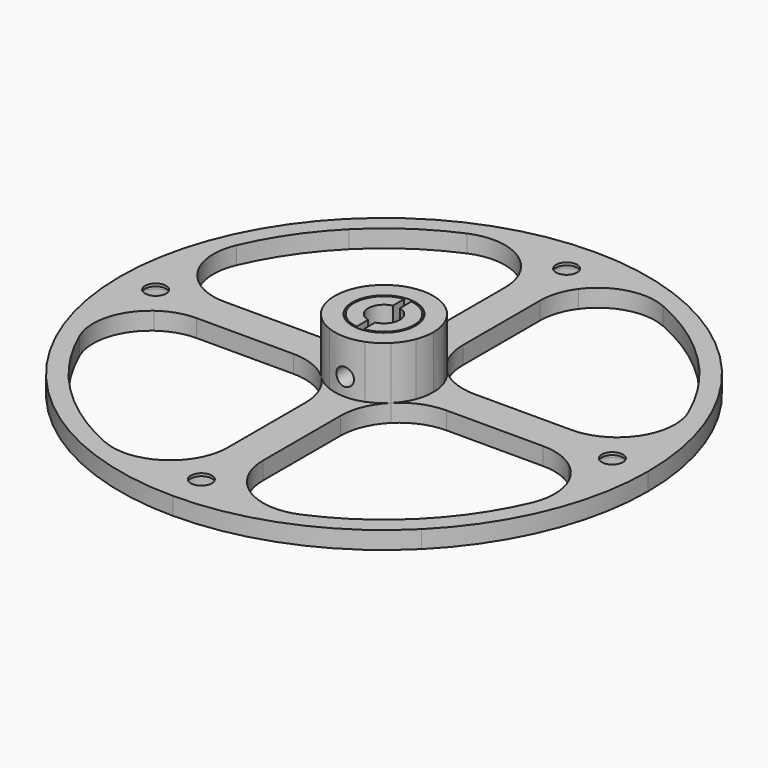
from build123d import *

# Parameters (mm, degrees)
F3_R          = 1.2
F3_R_2        = 2.05
F4_DEPTH      = 1
F4_DEPTH_BACK = 1
F5_DEPTH      = 1
F5_DEPTH_BACK = 1
F6_DEPTH      = 7
F7_DEPTH      = 0.7
F7_DEPTH_BACK = 0.7
F8_R          = 1
F9_DEPTH      = 30
F9_DEPTH_BACK = 30
F11_DEPTH     = 8


with BuildPart() as f4:
    # F3 (on Top) → F4 (new body, two sides)
    with BuildSketch(Plane.XY) as f4_sk:
        with BuildLine():
            Line((-19.79899, 19.79899), (-21.213203, 21.213203))
            ThreePointArc((-21.213203, 21.213203), (-27.716386, 11.480503), (-30, 0))
            ThreePointArc((-30, 0), (-29.396228, 2.127442), (-27.764933, 3.620569))
            ThreePointArc((-27.764933, 3.620569), (-26.989532, 7.454205), (-25.687491, 11.142389))
            ThreePointArc((-25.687491, 11.142389), (-23.15144, 15.74836), (-19.79899, 19.79899))
        make_face()
        with BuildLine():
            ThreePointArc((-30, 0), (-27.716386, -11.480503), (-21.213203, -21.213203))
            Line((-21.213203, -21.213203), (-19.79899, -19.79899))
            ThreePointArc((-19.79899, -19.79899), (-23.15144, -15.74836), (-25.687491, -11.142389))
            ThreePointArc((-25.687491, -11.142389), (-26.989532, -7.454205), (-27.764933, -3.620569))
            ThreePointArc((-27.764933, -3.620569), (-29.396228, -2.127443), (-30, 0))
        make_face()
        with BuildLine():
            ThreePointArc((-23.555055, -3.265997), (-25.610097, -4.035711), (-27.764933, -3.620569))
            ThreePointArc((-27.764933, -3.620569), (-26.989532, -7.454205), (-25.687491, -11.142389))
            ThreePointArc((-25.687491, -11.142389), (-26.000354, -6.830824), (-23.555055, -3.265997))
        make_face()
        with BuildLine():
            Line((-19.687728, 2), (-22.428282, 2))
            ThreePointArc((-22.428282, 2), (-22.034297, 1.034297), (-21.9, 0))
            ThreePointArc((-21.9, 0), (-22.034297, -1.034297), (-22.428282, -2))
            Line((-22.428282, -2), (-19.687728, -2))
            Line((-19.687728, -2), (-8.691169, -2))
            Line((-8.691169, -2), (-5.230679, -2))
            ThreePointArc((-5.230679, -2), (-5.6, 0), (-5.230679, 2))
            Line((-5.230679, 2), (-8.691169, 2))
            Line((-8.691169, 2), (-19.687728, 2))
        make_face()
        with BuildLine():
            ThreePointArc((22.428282, -2), (21.9, 0), (22.428282, 2))
            Line((22.428282, 2), (19.687728, 2))
            Line((19.687728, 2), (8.691169, 2))
            Line((8.691169, 2), (5.230679, 2))
            ThreePointArc((5.230679, 2), (5.506896, 1.016907), (5.6, 0))
            ThreePointArc((5.6, 0), (5.506896, -1.016907), (5.230679, -2))
            Line((5.230679, -2), (8.691169, -2))
            Line((8.691169, -2), (19.687728, -2))
            Line((19.687728, -2), (22.428282, -2))
        make_face()
        with BuildLine():
            Line((-2, -8.691169), (-2, -19.687728))
            Line((-2, -19.687728), (-2, -22.428282))
            ThreePointArc((-2, -22.428282), (0, -21.9), (2, -22.428282))
            Line((2, -22.428282), (2, -19.687728))
            Line((2, -19.687728), (2, -8.691169))
            Line((2, -8.691169), (2, -5.230679))
            ThreePointArc((2, -5.230679), (0, -5.6), (-2, -5.230679))
            Line((-2, -5.230679), (-2, -8.691169))
        make_face()
        with BuildLine():
            ThreePointArc((2, 22.428282), (0, 21.9), (-2, 22.428282))
            Line((-2, 22.428282), (-2, 19.687728))
            Line((-2, 19.687728), (-2, 8.691169))
            Line((-2, 8.691169), (-2, 5.230679))
            ThreePointArc((-2, 5.230679), (0, 5.6), (2, 5.230679))
            Line((2, 5.230679), (2, 8.691169))
            Line((2, 8.691169), (2, 19.687728))
            Line((2, 19.687728), (2, 22.428282))
        make_face()
        with BuildLine():
            ThreePointArc((-3.620569, 27.764933), (-2.127442, 29.396228), (0, 30))
            ThreePointArc((0, 30), (-11.480503, 27.716386), (-21.213203, 21.213203))
            Line((-21.213203, 21.213203), (-19.79899, 19.79899))
            ThreePointArc((-19.79899, 19.79899), (-15.74836, 23.15144), (-11.142389, 25.687491))
            ThreePointArc((-11.142389, 25.687491), (-7.454205, 26.989532), (-3.620569, 27.764933))
        make_face()
        with BuildLine():
            Line((19.79899, 19.79899), (21.213203, 21.213203))
            ThreePointArc((21.213203, 21.213203), (11.480503, 27.716386), (0, 30))
            ThreePointArc((0, 30), (2.127442, 29.396228), (3.620569, 27.764933))
            ThreePointArc((3.620569, 27.764933), (7.454205, 26.989532), (11.142389, 25.687491))
            ThreePointArc((11.142389, 25.687491), (15.74836, 23.15144), (19.79899, 19.79899))
        make_face()
        with BuildLine():
            ThreePointArc((3.620569, 27.764933), (2.127442, 29.396228), (0, 30))
            ThreePointArc((0, 30), (-2.127442, 29.396228), (-3.620569, 27.764933))
            ThreePointArc((-3.620569, 27.764933), (-1.814096, 27.941171), (0, 28))
            ThreePointArc((0, 28), (1.814096, 27.941171), (3.620569, 27.764933))
        make_face()
        with BuildLine():
            ThreePointArc((4.05, 25.95), (3.94118, 26.882522), (3.620569, 27.764933))
            ThreePointArc((3.620569, 27.764933), (1.814096, 27.941171), (0, 28))
            ThreePointArc((0, 28), (-1.814096, 27.941171), (-3.620569, 27.764933))
            ThreePointArc((-3.620569, 27.764933), (-4.035711, 25.610097), (-3.265997, 23.555055))
            ThreePointArc((-3.265997, 23.555055), (-2.692599, 22.924704), (-2, 22.428282))
            ThreePointArc((-2, 22.428282), (0, 21.9), (2, 22.428282))
            ThreePointArc((2, 22.428282), (2.692599, 22.924704), (3.265997, 23.555055))
            ThreePointArc((3.265997, 23.555055), (3.849012, 24.689998), (4.05, 25.95))
        make_face()
        with BuildLine():
            ThreePointArc((2.05, 25.95), (-1.449569, 24.500431), (0, 28))
            ThreePointArc((0, 28), (1.449569, 27.399569), (2.05, 25.95))
        make_face(mode=Mode.SUBTRACT)
        with BuildLine():
            ThreePointArc((-23.555055, 3.265998), (-25.610097, 4.035711), (-27.764933, 3.620569))
            ThreePointArc((-27.764933, 3.620569), (-27.941171, 1.814096), (-28, 0))
            ThreePointArc((-28, 0), (-27.941171, -1.814096), (-27.764933, -3.620569))
            ThreePointArc((-27.764933, -3.620569), (-25.610097, -4.035711), (-23.555055, -3.265997))
            ThreePointArc((-23.555055, -3.265997), (-22.924704, -2.692599), (-22.428282, -2))
            ThreePointArc((-22.428282, -2), (-22.034297, -1.034297), (-21.9, 0))
            ThreePointArc((-21.9, 0), (-22.034297, 1.034297), (-22.428282, 2))
            ThreePointArc((-22.428282, 2), (-22.924705, 2.692599), (-23.555055, 3.265998))
        make_face()
        with BuildLine():
            ThreePointArc((-23.9, 0), (-25.95, -2.05), (-28, 0))
            ThreePointArc((-28, 0), (-25.95, 2.05), (-23.9, 0))
        make_face(mode=Mode.SUBTRACT)
        with BuildLine():
            ThreePointArc((-27.764933, 3.620569), (-29.396228, 2.127442), (-30, 0))
            ThreePointArc((-30, 0), (-29.396228, -2.127443), (-27.764933, -3.620569))
            ThreePointArc((-27.764933, -3.620569), (-27.941171, -1.814096), (-28, 0))
            ThreePointArc((-28, 0), (-27.941171, 1.814096), (-27.764933, 3.620569))
        make_face()
        with BuildLine():
            ThreePointArc((-23.9, 0), (-25.95, 2.05), (-28, 0))
            ThreePointArc((-28, 0), (-25.95, -2.05), (-23.9, 0))
        make_face()
        with Locations((-25.95, 0)):
            Circle(F3_R, mode=Mode.SUBTRACT)
        with BuildLine():
            ThreePointArc((0, -30), (11.480503, -27.716386), (21.213203, -21.213203))
            Line((21.213203, -21.213203), (19.79899, -19.79899))
            ThreePointArc((19.79899, -19.79899), (15.74836, -23.15144), (11.142389, -25.687491))
            ThreePointArc((11.142389, -25.687491), (7.454205, -26.989532), (3.620569, -27.764933))
            ThreePointArc((3.620569, -27.764933), (2.127442, -29.396228), (0, -30))
        make_face()
        with BuildLine():
            ThreePointArc((-21.213203, -21.213203), (-11.480503, -27.716386), (0, -30))
            ThreePointArc((0, -30), (-2.127443, -29.396228), (-3.620569, -27.764933))
            ThreePointArc((-3.620569, -27.764933), (-7.454205, -26.989532), (-11.142389, -25.687491))
            ThreePointArc((-11.142389, -25.687491), (-15.74836, -23.15144), (-19.79899, -19.79899))
            Line((-19.79899, -19.79899), (-21.213203, -21.213203))
        make_face()
        with BuildLine():
            ThreePointArc((-3.265998, -23.555055), (-4.035711, -25.610097), (-3.620569, -27.764933))
            ThreePointArc((-3.620569, -27.764933), (-1.814096, -27.941171), (0, -28))
            ThreePointArc((0, -28), (1.814096, -27.941171), (3.620569, -27.764933))
            ThreePointArc((3.620569, -27.764933), (3.94118, -26.882522), (4.05, -25.95))
            ThreePointArc((4.05, -25.95), (3.849012, -24.689998), (3.265997, -23.555055))
            ThreePointArc((3.265997, -23.555055), (2.692599, -22.924704), (2, -22.428282))
            ThreePointArc((2, -22.428282), (0, -21.9), (-2, -22.428282))
            ThreePointArc((-2, -22.428282), (-2.692599, -22.924704), (-3.265998, -23.555055))
        make_face()
        with BuildLine():
            ThreePointArc((2.05, -25.95), (1.449569, -27.399569), (0, -28))
            ThreePointArc((0, -28), (-1.449569, -24.500431), (2.05, -25.95))
        make_face(mode=Mode.SUBTRACT)
        with BuildLine():
            ThreePointArc((-3.620569, -27.764933), (-2.127443, -29.396228), (0, -30))
            ThreePointArc((0, -30), (2.127442, -29.396228), (3.620569, -27.764933))
            ThreePointArc((3.620569, -27.764933), (1.814096, -27.941171), (0, -28))
            ThreePointArc((0, -28), (-1.814096, -27.941171), (-3.620569, -27.764933))
        make_face()
        with BuildLine():
            ThreePointArc((28, 0), (27.941171, 1.814096), (27.764933, 3.620569))
            ThreePointArc((27.764933, 3.620569), (25.610097, 4.035711), (23.555055, 3.265998))
            ThreePointArc((23.555055, 3.265998), (22.924704, 2.692599), (22.428282, 2))
            ThreePointArc((22.428282, 2), (21.9, 0), (22.428282, -2))
            ThreePointArc((22.428282, -2), (22.924705, -2.692599), (23.555055, -3.265998))
            ThreePointArc((23.555055, -3.265998), (25.610097, -4.035711), (27.764933, -3.620569))
            ThreePointArc((27.764933, -3.620569), (27.941171, -1.814096), (28, 0))
        make_face()
        with Locations((25.95, 0)):
            Circle(F3_R_2, mode=Mode.SUBTRACT)
        with BuildLine():
            ThreePointArc((27.764933, -3.620569), (29.396228, -2.127442), (30, 0))
            ThreePointArc((30, 0), (29.396228, 2.127442), (27.764933, 3.620569))
            ThreePointArc((27.764933, 3.620569), (27.941171, 1.814096), (28, 0))
            ThreePointArc((28, 0), (27.941171, -1.814096), (27.764933, -3.620569))
        make_face()
        with BuildLine():
            ThreePointArc((2.05, 25.95), (1.449569, 27.399569), (0, 28))
            ThreePointArc((0, 28), (-1.449569, 24.500431), (2.05, 25.95))
        make_face()
        with Locations((0, 25.95)):
            Circle(F3_R, mode=Mode.SUBTRACT)
        with BuildLine():
            ThreePointArc((2.05, -25.95), (-1.449569, -24.500431), (0, -28))
            ThreePointArc((0, -28), (1.449569, -27.399569), (2.05, -25.95))
        make_face()
        with Locations((0, -25.95)):
            Circle(F3_R, mode=Mode.SUBTRACT)
        with Locations((25.95, 0)):
            Circle(F3_R_2)
        with Locations((25.95, 0)):
            Circle(F3_R, mode=Mode.SUBTRACT)
        with BuildLine():
            ThreePointArc((21.213203, -21.213203), (27.716386, -11.480503), (30, 0))
            ThreePointArc((30, 0), (29.396228, -2.127442), (27.764933, -3.620569))
            ThreePointArc((27.764933, -3.620569), (26.989532, -7.454205), (25.687491, -11.142389))
            ThreePointArc((25.687491, -11.142389), (23.15144, -15.74836), (19.79899, -19.79899))
            Line((19.79899, -19.79899), (21.213203, -21.213203))
        make_face()
        with BuildLine():
            ThreePointArc((27.764933, 3.620569), (29.396228, 2.127442), (30, 0))
            ThreePointArc((30, 0), (27.716386, 11.480503), (21.213203, 21.213203))
            Line((21.213203, 21.213203), (19.79899, 19.79899))
            ThreePointArc((19.79899, 19.79899), (23.15144, 15.74836), (25.687491, 11.142389))
            ThreePointArc((25.687491, 11.142389), (26.989532, 7.454205), (27.764933, 3.620569))
        make_face()
        with BuildLine():
            ThreePointArc((5.230679, 2), (4.698555, 3.046897), (3.959798, 3.959798))
            Line((3.959798, 3.959798), (2.545584, 2.545584))
            ThreePointArc((2.545584, 2.545584), (3.325966, 1.37766), (3.6, 0))
            ThreePointArc((3.6, 0), (3.325966, -1.37766), (2.545584, -2.545584))
            Line((2.545584, -2.545584), (3.959798, -3.959798))
            ThreePointArc((3.959798, -3.959798), (4.698555, -3.046897), (5.230679, -2))
            ThreePointArc((5.230679, -2), (5.506896, -1.016907), (5.6, 0))
            ThreePointArc((5.6, 0), (5.506896, 1.016907), (5.230679, 2))
        make_face()
        with BuildLine():
            Line((2.545584, 2.545584), (3.959798, 3.959798))
            ThreePointArc((3.959798, 3.959798), (3.046897, 4.698555), (2, 5.230679))
            ThreePointArc((2, 5.230679), (0, 5.6), (-2, 5.230679))
            ThreePointArc((-2, 5.230679), (-3.046897, 4.698555), (-3.959798, 3.959798))
            Line((-3.959798, 3.959798), (-2.545584, 2.545584))
            ThreePointArc((-2.545584, 2.545584), (0, 3.6), (2.545584, 2.545584))
        make_face()
        with BuildLine():
            Line((-2.545584, 2.545584), (-3.959798, 3.959798))
            ThreePointArc((-3.959798, 3.959798), (-4.698555, 3.046897), (-5.230679, 2))
            ThreePointArc((-5.230679, 2), (-5.6, 0), (-5.230679, -2))
            ThreePointArc((-5.230679, -2), (-4.698555, -3.046897), (-3.959798, -3.959798))
            Line((-3.959798, -3.959798), (-2.545584, -2.545584))
            ThreePointArc((-2.545584, -2.545584), (-3.6, 0), (-2.545584, 2.545584))
        make_face()
        with BuildLine():
            ThreePointArc((2, -5.230679), (3.046897, -4.698555), (3.959798, -3.959798))
            Line((3.959798, -3.959798), (2.545584, -2.545584))
            ThreePointArc((2.545584, -2.545584), (0, -3.6), (-2.545584, -2.545584))
            Line((-2.545584, -2.545584), (-3.959798, -3.959798))
            ThreePointArc((-3.959798, -3.959798), (-3.046897, -4.698555), (-2, -5.230679))
            ThreePointArc((-2, -5.230679), (0, -5.6), (2, -5.230679))
        make_face()
        with BuildLine():
            ThreePointArc((-2.545584, -2.545584), (0, -3.6), (2.545584, -2.545584))
            Line((2.545584, -2.545584), (1.131371, -1.131371))
            ThreePointArc((1.131371, -1.131371), (0, -1.6), (-1.131371, -1.131371))
            Line((-1.131371, -1.131371), (-2.545584, -2.545584))
        make_face()
        with BuildLine():
            ThreePointArc((3.6, 0), (3.325966, 1.37766), (2.545584, 2.545584))
            Line((2.545584, 2.545584), (1.131371, 1.131371))
            ThreePointArc((1.131371, 1.131371), (1.478207, 0.612293), (1.6, 0))
            ThreePointArc((1.6, 0), (1.478207, -0.612293), (1.131371, -1.131371))
            Line((1.131371, -1.131371), (2.545584, -2.545584))
            ThreePointArc((2.545584, -2.545584), (3.325966, -1.37766), (3.6, 0))
        make_face()
        with BuildLine():
            Line((1.131371, 1.131371), (2.545584, 2.545584))
            ThreePointArc((2.545584, 2.545584), (0, 3.6), (-2.545584, 2.545584))
            Line((-2.545584, 2.545584), (-1.131371, 1.131371))
            ThreePointArc((-1.131371, 1.131371), (0, 1.6), (1.131371, 1.131371))
        make_face()
        with BuildLine():
            Line((-1.131371, 1.131371), (-2.545584, 2.545584))
            ThreePointArc((-2.545584, 2.545584), (-3.6, 0), (-2.545584, -2.545584))
            Line((-2.545584, -2.545584), (-1.131371, -1.131371))
            ThreePointArc((-1.131371, -1.131371), (-1.6, 0), (-1.131371, 1.131371))
        make_face()
        with BuildLine():
            Line((0, 0), (-1.131371, 1.131371))
            ThreePointArc((-1.131371, 1.131371), (-1.6, 0), (-1.131371, -1.131371))
            Line((-1.131371, -1.131371), (0, 0))
        make_face()
        with BuildLine():
            Line((0, 0), (1.131371, 1.131371))
            ThreePointArc((1.131371, 1.131371), (0, 1.6), (-1.131371, 1.131371))
            Line((-1.131371, 1.131371), (0, 0))
        make_face()
        with BuildLine():
            ThreePointArc((1.6, 0), (1.478207, 0.612293), (1.131371, 1.131371))
            Line((1.131371, 1.131371), (0, 0))
            Line((0, 0), (1.131371, -1.131371))
            ThreePointArc((1.131371, -1.131371), (1.478207, -0.612293), (1.6, 0))
        make_face()
        with BuildLine():
            ThreePointArc((-1.131371, -1.131371), (0, -1.6), (1.131371, -1.131371))
            Line((1.131371, -1.131371), (0, 0))
            Line((0, 0), (-1.131371, -1.131371))
        make_face()
        with BuildLine():
            ThreePointArc((-5.230679, 2), (-4.698555, 3.046897), (-3.959798, 3.959798))
            ThreePointArc((-3.959798, 3.959798), (-6.130569, 2.509335), (-8.691169, 2))
            Line((-8.691169, 2), (-5.230679, 2))
        make_face()
        with BuildLine():
            ThreePointArc((-2, 8.691169), (-2.509335, 6.130569), (-3.959798, 3.959798))
            ThreePointArc((-3.959798, 3.959798), (-3.046897, 4.698555), (-2, 5.230679))
            Line((-2, 5.230679), (-2, 8.691169))
        make_face()
        with BuildLine():
            ThreePointArc((-25.687491, 11.142389), (-26.989532, 7.454205), (-27.764933, 3.620569))
            ThreePointArc((-27.764933, 3.620569), (-25.610097, 4.035711), (-23.555055, 3.265998))
            ThreePointArc((-23.555055, 3.265998), (-26.000354, 6.830824), (-25.687491, 11.142389))
        make_face()
        with BuildLine():
            ThreePointArc((-19.687728, 2), (-21.722364, 2.324553), (-23.555055, 3.265998))
            ThreePointArc((-23.555055, 3.265998), (-22.924705, 2.692599), (-22.428282, 2))
            Line((-22.428282, 2), (-19.687728, 2))
        make_face()
        with BuildLine():
            ThreePointArc((-3.265997, 23.555055), (-4.035711, 25.610097), (-3.620569, 27.764933))
            ThreePointArc((-3.620569, 27.764933), (-7.454205, 26.989532), (-11.142389, 25.687491))
            ThreePointArc((-11.142389, 25.687491), (-6.830824, 26.000354), (-3.265997, 23.555055))
        make_face()
        with BuildLine():
            ThreePointArc((-2, 22.428282), (-2.692599, 22.924704), (-3.265997, 23.555055))
            ThreePointArc((-3.265997, 23.555055), (-2.324553, 21.722364), (-2, 19.687728))
            Line((-2, 19.687728), (-2, 22.428282))
        make_face()
        with BuildLine():
            ThreePointArc((11.142389, 25.687491), (7.454205, 26.989532), (3.620569, 27.764933))
            ThreePointArc((3.620569, 27.764933), (3.94118, 26.882522), (4.05, 25.95))
            ThreePointArc((4.05, 25.95), (3.849012, 24.689998), (3.265997, 23.555055))
            ThreePointArc((3.265997, 23.555055), (6.830824, 26.000354), (11.142389, 25.687491))
        make_face()
        with BuildLine():
            ThreePointArc((2, 19.687728), (2.324553, 21.722364), (3.265997, 23.555055))
            ThreePointArc((3.265997, 23.555055), (2.692599, 22.924704), (2, 22.428282))
            Line((2, 22.428282), (2, 19.687728))
        make_face()
        with BuildLine():
            ThreePointArc((23.555055, 3.265998), (25.610097, 4.035711), (27.764933, 3.620569))
            ThreePointArc((27.764933, 3.620569), (26.989532, 7.454205), (25.687491, 11.142389))
            ThreePointArc((25.687491, 11.142389), (26.091162, 9.868868), (26.227618, 8.539889))
            ThreePointArc((26.227618, 8.539889), (25.52134, 5.583687), (23.555055, 3.265998))
        make_face()
        with BuildLine():
            ThreePointArc((22.428282, 2), (22.924704, 2.692599), (23.555055, 3.265998))
            ThreePointArc((23.555055, 3.265998), (21.722364, 2.324553), (19.687728, 2))
            Line((19.687728, 2), (22.428282, 2))
        make_face()
        with BuildLine():
            ThreePointArc((8.691169, 2), (6.130569, 2.509335), (3.959798, 3.959798))
            ThreePointArc((3.959798, 3.959798), (4.698555, 3.046897), (5.230679, 2))
            Line((5.230679, 2), (8.691169, 2))
        make_face()
        with BuildLine():
            ThreePointArc((2, 5.230679), (3.046897, 4.698555), (3.959798, 3.959798))
            ThreePointArc((3.959798, 3.959798), (2.509335, 6.130569), (2, 8.691169))
            Line((2, 8.691169), (2, 5.230679))
        make_face()
        with BuildLine():
            ThreePointArc((-22.428282, -2), (-22.924704, -2.692599), (-23.555055, -3.265997))
            ThreePointArc((-23.555055, -3.265997), (-21.722364, -2.324553), (-19.687728, -2))
            Line((-19.687728, -2), (-22.428282, -2))
        make_face()
        with BuildLine():
            ThreePointArc((-8.691169, -2), (-6.130569, -2.509335), (-3.959798, -3.959798))
            ThreePointArc((-3.959798, -3.959798), (-4.698555, -3.046897), (-5.230679, -2))
            Line((-5.230679, -2), (-8.691169, -2))
        make_face()
        with BuildLine():
            ThreePointArc((-2, -5.230679), (-3.046897, -4.698555), (-3.959798, -3.959798))
            ThreePointArc((-3.959798, -3.959798), (-2.509335, -6.130569), (-2, -8.691169))
            Line((-2, -8.691169), (-2, -5.230679))
        make_face()
        with BuildLine():
            ThreePointArc((-11.142389, -25.687491), (-7.454205, -26.989532), (-3.620569, -27.764933))
            ThreePointArc((-3.620569, -27.764933), (-4.035711, -25.610097), (-3.265998, -23.555055))
            ThreePointArc((-3.265998, -23.555055), (-6.830824, -26.000354), (-11.142389, -25.687491))
        make_face()
        with BuildLine():
            ThreePointArc((-2, -19.687728), (-2.324553, -21.722364), (-3.265998, -23.555055))
            ThreePointArc((-3.265998, -23.555055), (-2.692599, -22.924704), (-2, -22.428282))
            Line((-2, -22.428282), (-2, -19.687728))
        make_face()
        with BuildLine():
            ThreePointArc((4.05, -25.95), (3.94118, -26.882522), (3.620569, -27.764933))
            ThreePointArc((3.620569, -27.764933), (7.454205, -26.989532), (11.142389, -25.687491))
            ThreePointArc((11.142389, -25.687491), (6.830824, -26.000354), (3.265997, -23.555055))
            ThreePointArc((3.265997, -23.555055), (3.849012, -24.689998), (4.05, -25.95))
        make_face()
        with BuildLine():
            ThreePointArc((2, -22.428282), (2.692599, -22.924704), (3.265997, -23.555055))
            ThreePointArc((3.265997, -23.555055), (2.324553, -21.722364), (2, -19.687728))
            Line((2, -19.687728), (2, -22.428282))
        make_face()
        with BuildLine():
            ThreePointArc((19.687728, -2), (21.722364, -2.324553), (23.555055, -3.265998))
            ThreePointArc((23.555055, -3.265998), (22.924705, -2.692599), (22.428282, -2))
            Line((22.428282, -2), (19.687728, -2))
        make_face()
        with BuildLine():
            ThreePointArc((25.687491, -11.142389), (26.989532, -7.454205), (27.764933, -3.620569))
            ThreePointArc((27.764933, -3.620569), (25.610097, -4.035711), (23.555055, -3.265998))
            ThreePointArc((23.555055, -3.265998), (25.52134, -5.583687), (26.227618, -8.539889))
            ThreePointArc((26.227618, -8.539889), (26.091162, -9.868868), (25.687491, -11.142389))
        make_face()
        with BuildLine():
            ThreePointArc((5.230679, -2), (4.698555, -3.046897), (3.959798, -3.959798))
            ThreePointArc((3.959798, -3.959798), (6.130569, -2.509335), (8.691169, -2))
            Line((8.691169, -2), (5.230679, -2))
        make_face()
        with BuildLine():
            ThreePointArc((2, -8.691169), (2.509335, -6.130569), (3.959798, -3.959798))
            ThreePointArc((3.959798, -3.959798), (3.046897, -4.698555), (2, -5.230679))
            Line((2, -5.230679), (2, -8.691169))
        make_face()
    extrude(amount=F4_DEPTH)
    extrude(f4_sk.sketch, amount=-F4_DEPTH_BACK)

    # F3 (on Top) → F5 (cut, two sides)
    with BuildSketch(Plane.XY) as f5_sk:
        with BuildLine():
            Line((0, 0), (1.131371, 1.131371))
            ThreePointArc((1.131371, 1.131371), (0, 1.6), (-1.131371, 1.131371))
            Line((-1.131371, 1.131371), (0, 0))
        make_face()
        with BuildLine():
            ThreePointArc((1.6, 0), (1.478207, 0.612293), (1.131371, 1.131371))
            Line((1.131371, 1.131371), (0, 0))
            Line((0, 0), (1.131371, -1.131371))
            ThreePointArc((1.131371, -1.131371), (1.478207, -0.612293), (1.6, 0))
        make_face()
        with BuildLine():
            ThreePointArc((-1.131371, -1.131371), (0, -1.6), (1.131371, -1.131371))
            Line((1.131371, -1.131371), (0, 0))
            Line((0, 0), (-1.131371, -1.131371))
        make_face()
        with BuildLine():
            Line((0, 0), (-1.131371, 1.131371))
            ThreePointArc((-1.131371, 1.131371), (-1.6, 0), (-1.131371, -1.131371))
            Line((-1.131371, -1.131371), (0, 0))
        make_face()
        with BuildLine():
            Line((-1.131371, 1.131371), (-2.545584, 2.545584))
            ThreePointArc((-2.545584, 2.545584), (-3.6, 0), (-2.545584, -2.545584))
            Line((-2.545584, -2.545584), (-1.131371, -1.131371))
            ThreePointArc((-1.131371, -1.131371), (-1.6, 0), (-1.131371, 1.131371))
        make_face()
        with BuildLine():
            Line((1.131371, 1.131371), (2.545584, 2.545584))
            ThreePointArc((2.545584, 2.545584), (0, 3.6), (-2.545584, 2.545584))
            Line((-2.545584, 2.545584), (-1.131371, 1.131371))
            ThreePointArc((-1.131371, 1.131371), (0, 1.6), (1.131371, 1.131371))
        make_face()
        with BuildLine():
            ThreePointArc((3.6, 0), (3.325966, 1.37766), (2.545584, 2.545584))
            Line((2.545584, 2.545584), (1.131371, 1.131371))
            ThreePointArc((1.131371, 1.131371), (1.478207, 0.612293), (1.6, 0))
            ThreePointArc((1.6, 0), (1.478207, -0.612293), (1.131371, -1.131371))
            Line((1.131371, -1.131371), (2.545584, -2.545584))
            ThreePointArc((2.545584, -2.545584), (3.325966, -1.37766), (3.6, 0))
        make_face()
        with BuildLine():
            ThreePointArc((-2.545584, -2.545584), (0, -3.6), (2.545584, -2.545584))
            Line((2.545584, -2.545584), (1.131371, -1.131371))
            ThreePointArc((1.131371, -1.131371), (0, -1.6), (-1.131371, -1.131371))
            Line((-1.131371, -1.131371), (-2.545584, -2.545584))
        make_face()
    extrude(amount=F5_DEPTH, mode=Mode.SUBTRACT)
    extrude(f5_sk.sketch, amount=-F5_DEPTH_BACK, mode=Mode.SUBTRACT)

    # F3 (on Top) → F6 (join)
    with BuildSketch(Plane.XY):
        with BuildLine():
            Line((2.545584, 2.545584), (3.959798, 3.959798))
            ThreePointArc((3.959798, 3.959798), (3.046897, 4.698555), (2, 5.230679))
            ThreePointArc((2, 5.230679), (0, 5.6), (-2, 5.230679))
            ThreePointArc((-2, 5.230679), (-3.046897, 4.698555), (-3.959798, 3.959798))
            Line((-3.959798, 3.959798), (-2.545584, 2.545584))
            ThreePointArc((-2.545584, 2.545584), (0, 3.6), (2.545584, 2.545584))
        make_face()
        with BuildLine():
            Line((-2.545584, 2.545584), (-3.959798, 3.959798))
            ThreePointArc((-3.959798, 3.959798), (-4.698555, 3.046897), (-5.230679, 2))
            ThreePointArc((-5.230679, 2), (-5.6, 0), (-5.230679, -2))
            ThreePointArc((-5.230679, -2), (-4.698555, -3.046897), (-3.959798, -3.959798))
            Line((-3.959798, -3.959798), (-2.545584, -2.545584))
            ThreePointArc((-2.545584, -2.545584), (-3.6, 0), (-2.545584, 2.545584))
        make_face()
        with BuildLine():
            ThreePointArc((2, -5.230679), (3.046897, -4.698555), (3.959798, -3.959798))
            Line((3.959798, -3.959798), (2.545584, -2.545584))
            ThreePointArc((2.545584, -2.545584), (0, -3.6), (-2.545584, -2.545584))
            Line((-2.545584, -2.545584), (-3.959798, -3.959798))
            ThreePointArc((-3.959798, -3.959798), (-3.046897, -4.698555), (-2, -5.230679))
            ThreePointArc((-2, -5.230679), (0, -5.6), (2, -5.230679))
        make_face()
        with BuildLine():
            ThreePointArc((5.230679, 2), (4.698555, 3.046897), (3.959798, 3.959798))
            Line((3.959798, 3.959798), (2.545584, 2.545584))
            ThreePointArc((2.545584, 2.545584), (3.325966, 1.37766), (3.6, 0))
            ThreePointArc((3.6, 0), (3.325966, -1.37766), (2.545584, -2.545584))
            Line((2.545584, -2.545584), (3.959798, -3.959798))
            ThreePointArc((3.959798, -3.959798), (4.698555, -3.046897), (5.230679, -2))
            ThreePointArc((5.230679, -2), (5.506896, -1.016907), (5.6, 0))
            ThreePointArc((5.6, 0), (5.506896, 1.016907), (5.230679, 2))
        make_face()
    extrude(amount=F6_DEPTH)

    # F3 (on Top) → F7 (cut, two sides)
    with BuildSketch(Plane.XY) as f7_sk:
        with BuildLine():
            ThreePointArc((-23.9, 0), (-25.95, 2.05), (-28, 0))
            ThreePointArc((-28, 0), (-25.95, -2.05), (-23.9, 0))
        make_face()
        with Locations((-25.95, 0)):
            Circle(F3_R, mode=Mode.SUBTRACT)
        with BuildLine():
            ThreePointArc((2.05, 25.95), (1.449569, 27.399569), (0, 28))
            ThreePointArc((0, 28), (-1.449569, 24.500431), (2.05, 25.95))
        make_face()
        with Locations((0, 25.95)):
            Circle(F3_R, mode=Mode.SUBTRACT)
        with Locations((25.95, 0)):
            Circle(F3_R_2)
        with Locations((25.95, 0)):
            Circle(F3_R, mode=Mode.SUBTRACT)
        with BuildLine():
            ThreePointArc((2.05, -25.95), (-1.449569, -24.500431), (0, -28))
            ThreePointArc((0, -28), (1.449569, -27.399569), (2.05, -25.95))
        make_face()
        with Locations((0, -25.95)):
            Circle(F3_R, mode=Mode.SUBTRACT)
    extrude(amount=-F7_DEPTH, mode=Mode.SUBTRACT)
    extrude(f7_sk.sketch, amount=F7_DEPTH_BACK, mode=Mode.SUBTRACT)

    # F8 (on Front) → F9 (cut, two sides)
    with BuildSketch(Plane.XZ) as f9_sk:
        with Locations((0, 3)):
            Circle(F8_R)
    extrude(amount=-F9_DEPTH, mode=Mode.SUBTRACT)
    extrude(f9_sk.sketch, amount=F9_DEPTH_BACK, mode=Mode.SUBTRACT)


with BuildPart() as f11:
    # F10 (on face) → F11 (new body)
    with BuildSketch(Plane(origin=(0, 0, -1), x_dir=(1, 0, 0), z_dir=(0, 0, -1))):
        with BuildLine():
            Line((-0.4, 1.754993), (-0.4, 3.376389))
            ThreePointArc((-0.4, 3.376389), (-3.4, 0), (-0.4, -3.376389))
            Line((-0.4, -3.376389), (-0.4, -1.754993))
            ThreePointArc((-0.4, -1.754993), (-1.8, 0), (-0.4, 1.754993))
        make_face()
    extrude(amount=-F11_DEPTH)


with BuildPart() as f11b:
    # F10 (on face) → F11, piece 2 (new body)
    with BuildSketch(Plane(origin=(0, 0, -1), x_dir=(1, 0, 0), z_dir=(0, 0, -1))):
        with BuildLine():
            ThreePointArc((0.4, -3.376389), (2.541653, -2.258318), (3.4, 0))
            ThreePointArc((3.4, 0), (2.541653, 2.258318), (0.4, 3.376389))
            Line((0.4, 3.376389), (0.4, 1.754993))
            ThreePointArc((0.4, 1.754993), (1.407125, 1.122497), (1.8, 0))
            ThreePointArc((1.8, 0), (1.407125, -1.122497), (0.4, -1.754993))
            Line((0.4, -1.754993), (0.4, -3.376389))
        make_face()
    extrude(amount=-F11_DEPTH)


solid = Compound([f4.part, f11.part, f11b.part])
